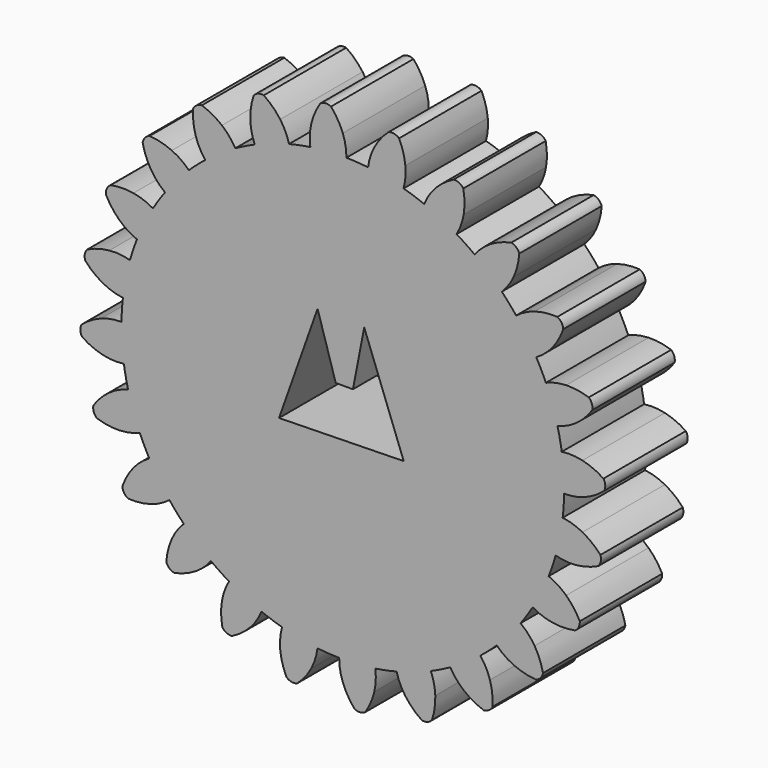
from build123d import *

# Parameters (mm, degrees)
F1_DEPTH = 25
F2_DEPTH = 25
F3_COUNT = 24
F4_DEPTH = 54.2


# Not quite as in the source:
# - a feature names something its author has since deleted; it is built from what else it names


with BuildPart() as f1:
    # F0 (on Front) → F1 (new body)
    with BuildSketch(Plane.XZ):
        with BuildLine():
            ThreePointArc((-7.8842675869, 53.139290225), (-35.0884247435, -40.6785974441), (53.721, 0))
            ThreePointArc((53.721, 0), (38.2966086664, 37.6738052983), (0.8807473744, 53.7137796572))
            ThreePointArc((0.8807473744, 53.7137796572), (-3.5135215054, 53.6059792153), (-7.8842675869, 53.139290225))
        make_face()
        Polygon((14.7791085765, -6.5843504854), (-15.4736051336, -7.2130695917), (-6.1205071397, 19.1956777126), (-1.7190492945, 4.7533949837), (2.4594513234, 4.7533949837), (5.1971534267, 18.876273185), align=None, mode=Mode.SUBTRACT)
    extrude(amount=F1_DEPTH)

    # F0 (on Front) → F2 (join)
    with BuildSketch(Plane.XZ):
        with BuildLine():
            ThreePointArc((-7.8842675869, 53.139290225), (-3.5135215054, 53.6059792153), (0.8807473744, 53.7137796572))
            ThreePointArc((0.8807473744, 53.7137796572), (0.6677080801, 56.2342558115), (0, 58.674))
            ThreePointArc((0, 58.674), (-1.2171778981, 61.1814598719), (-2.8564405638, 63.4357213824))
            ThreePointArc((-2.8564405638, 63.4357213824), (-4.1751502487, 63.70048315), (-5.448019844, 63.2658603022))
            ThreePointArc((-5.448019844, 63.2658603022), (-6.7790182191, 60.8169175976), (-7.6584938023, 58.1720357962))
            ThreePointArc((-7.6584938023, 58.1720357962), (-8.0020390283, 55.6660105643), (-7.8842675869, 53.139290225))
        make_face()
    extrude(amount=F2_DEPTH)

    # F3: F1 ×24 about axis
    f3_axis = Axis((0, 0, 0), (0, 1, 0))


with BuildPart() as f1_1:
    add(f1.part)
    for i in range(1, F3_COUNT):
        add(f1.part.rotate(f3_axis, i * 360 / F3_COUNT))

    # F0 (on Front) → F4 (cut)
    with BuildSketch(Plane.XZ):
        Polygon((-6.1205071397, 19.1956777126), (-15.4736051336, -7.2130695917), (14.7791085765, -6.5843504854), (5.1971534267, 18.876273185), (2.4594513234, 4.7533949837), (-1.7190492945, 4.7533949837), align=None)
    extrude(amount=F4_DEPTH, mode=Mode.SUBTRACT)


solid = f1_1.part
